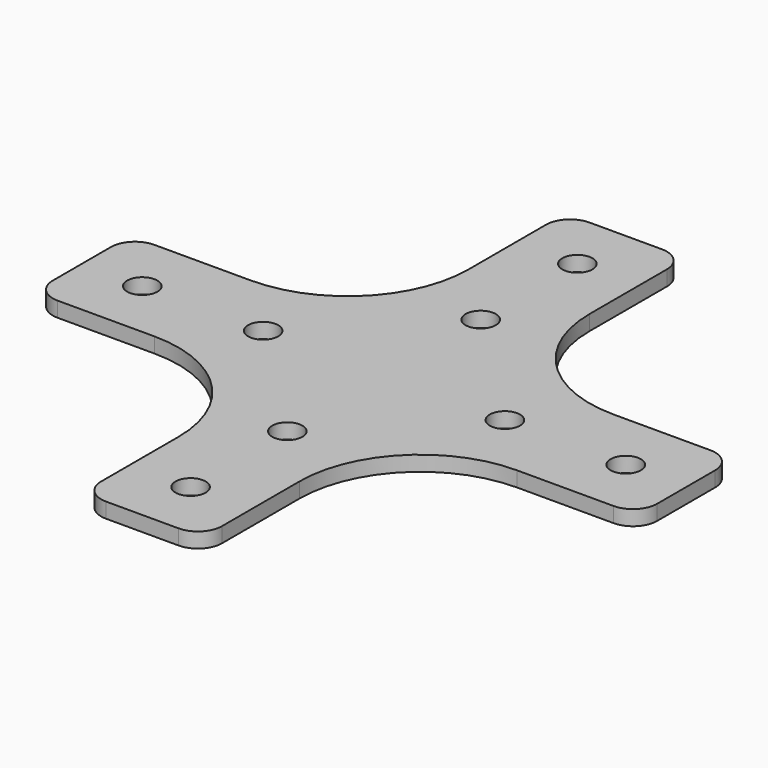
from build123d import *

# Parameters (mm, degrees)
F0_R     = 3.175
F1_DEPTH = 3.175


# Not quite as in the source:
# - a length typed as a fraction of an inch, garbled in the dataset ("3 / 203.2 mm" for 3/8 in), is restored


with BuildPart() as f1:
    # F0 (on Top) → F1 (new body)
    with BuildSketch(Plane.XY):
        with BuildLine():
            ThreePointArc((-63.5, -7.62), (-62.0121024484, -11.2121024484), (-58.42, -12.7))
            Line((-58.42, -12.7), (-38.1, -12.7))
            ThreePointArc((-38.1, -12.7), (-20.1394877579, -20.1394877579), (-12.7, -38.1))
            Line((-12.7, -38.1), (-12.7, -58.42))
            ThreePointArc((-12.7, -58.42), (-11.2121024484, -62.0121024484), (-7.62, -63.5))
            Line((-7.62, -63.5), (0, -63.5))
            Line((0, -63.5), (7.62, -63.5))
            ThreePointArc((7.62, -63.5), (11.2121024484, -62.0121024484), (12.7, -58.42))
            Line((12.7, -58.42), (12.7, -38.1))
            ThreePointArc((12.7, -38.1), (20.1394877579, -20.1394877579), (38.1, -12.7))
            Line((38.1, -12.7), (58.42, -12.7))
            ThreePointArc((58.42, -12.7), (62.0121024484, -11.2121024484), (63.5, -7.62))
            Line((63.5, -7.62), (63.5, 0))
            Line((63.5, 0), (63.5, 7.62))
            ThreePointArc((63.5, 7.62), (62.0121024484, 11.2121024484), (58.42, 12.7))
            Line((58.42, 12.7), (38.1, 12.7))
            ThreePointArc((38.1, 12.7), (20.1394877579, 20.1394877579), (12.7, 38.1))
            Line((12.7, 38.1), (12.7, 58.42))
            ThreePointArc((12.7, 58.42), (11.2121024484, 62.0121024484), (7.62, 63.5))
            Line((7.62, 63.5), (-7.62, 63.5))
            ThreePointArc((-7.62, 63.5), (-11.2121024484, 62.0121024484), (-12.7, 58.42))
            Line((-12.7, 58.42), (-12.7, 38.1))
            ThreePointArc((-12.7, 38.1), (-20.1394877579, 20.1394877579), (-38.1, 12.7))
            Line((-38.1, 12.7), (-58.42, 12.7))
            ThreePointArc((-58.42, 12.7), (-62.0121024484, 11.2121024484), (-63.5, 7.62))
            Line((-63.5, 7.62), (-63.5, 0))
            Line((-63.5, 0), (-63.5, -7.62))
        make_face()
        with Locations((0, -50.8)):
            Circle(F0_R, mode=Mode.SUBTRACT)
        with Locations((0, -25.4)):
            Circle(F0_R, mode=Mode.SUBTRACT)
        with Locations((-50.8, 0)):
            Circle(F0_R, mode=Mode.SUBTRACT)
        with Locations((-25.4, 0)):
            Circle(F0_R, mode=Mode.SUBTRACT)
        with Locations((25.4, 0)):
            Circle(F0_R, mode=Mode.SUBTRACT)
        with Locations((0, 25.4)):
            Circle(F0_R, mode=Mode.SUBTRACT)
        with Locations((50.8, 0)):
            Circle(F0_R, mode=Mode.SUBTRACT)
        with Locations((0, 50.8)):
            Circle(F0_R, mode=Mode.SUBTRACT)
    extrude(amount=F1_DEPTH)


solid = f1.part
